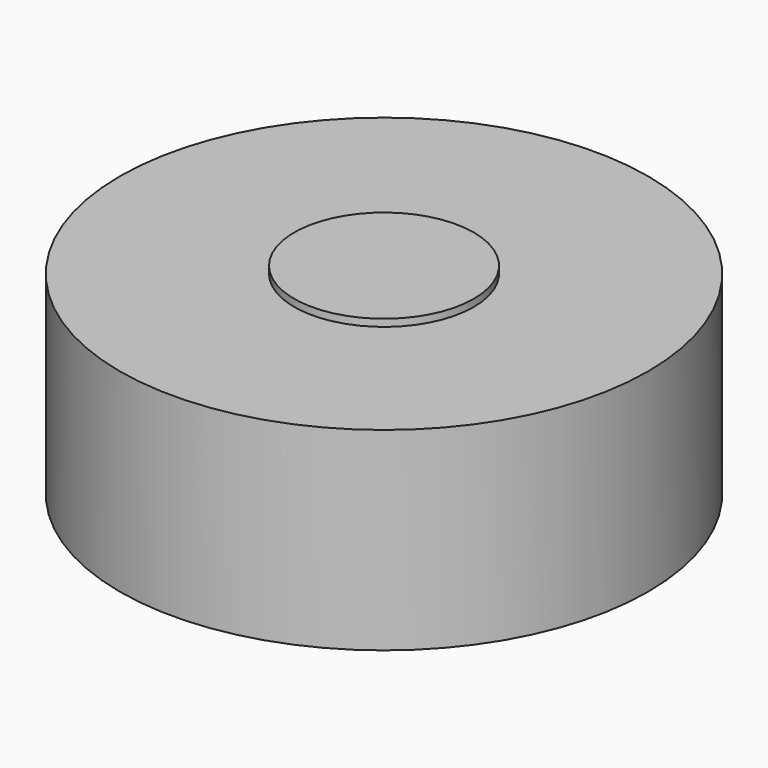
from build123d import *

# Parameters (mm, degrees)
F0_R        = 36.75
F0_R_2      = 30.75
F1_DEPTH    = 40
F2_START    = 20
F0_R_3      = 12.5
F2_DEPTH    = 20
F3_START    = 39
F3_DEPTH    = 2
F4_S5_R     = 30.75
F4_T6_DEPTH = 47
F5_DEPTH    = 13


# Not quite as in the source:
# - a fillet or chamfer that OpenCascade refuses, or shapes differently, is made with other operations: its cross-section is extruded or revolved along the edge and cut away or added


with BuildPart() as f1:
    # F0 (on Top) → F1 (new body)
    with BuildSketch(Plane.XY):
        Circle(F0_R)
        Circle(F0_R_2, mode=Mode.SUBTRACT)
    extrude(amount=F1_DEPTH)

    # F0 (on Top) → F2 (join)
    with BuildSketch(Plane.XY.offset(F2_START)):
        Circle(F0_R_2)
        Circle(F0_R_3, mode=Mode.SUBTRACT)
    extrude(amount=F2_DEPTH)

    # F0 (on Top) → F3 (join)
    with BuildSketch(Plane.XY.offset(F3_START)):
        Circle(F0_R_3)
    extrude(amount=F3_DEPTH)

    # F4: chamfer of 19 on 1 edges, made by hand


with BuildPart() as f4_tool2:
    # F4_s3 → F4_t4 (revolve)
    with BuildSketch(Plane.XZ):
        Polygon((31.5, 20), (12.5, 39), (12.5, 20), align=None)
    revolve(axis=Axis((0, 0, 20), (0, 0, 1)))

    # F4_s5 → F4_t6 (intersect, symmetric)
    with BuildSketch(Plane.XY.offset(29.5)):
        Circle(F4_S5_R)
    extrude(amount=F4_T6_DEPTH, both=True, mode=Mode.INTERSECT)

    split(bisect_by=Plane.XY.offset(39), keep=Keep.BOTTOM)


with BuildPart() as f1_1:
    add(f1.part)

    # F4_t1: cut F4_tool2
    add(f4_tool2.part, mode=Mode.SUBTRACT)

    # F5 (cut): a face of the model
    f5_faces = [f1_1.faces().sort_by_distance(p)[0] for p in [
        (-35.7105530317, 0, 0),
    ]]
    extrude(f5_faces, amount=-F5_DEPTH, mode=Mode.SUBTRACT)


solid = f1_1.part
